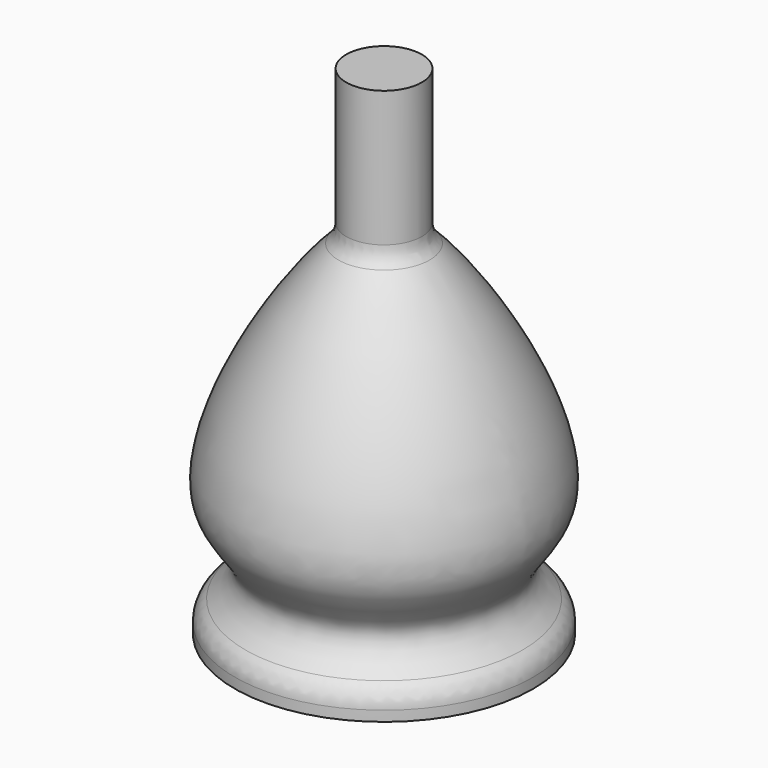
from build123d import *

# Parameters (mm, degrees)
F2_R     = 5.08
F3_DEPTH = 30.48
F4_R     = 5.08


with BuildPart() as f1:
    # F0 (on Front) → F1 (revolve)
    with BuildSketch(Plane.XZ):
        with BuildLine():
            add(Edge.make_bspline(
                [(8.1309033558, 71.12), (7.9376181833, 71.2042943301), (7.8304224666, 71.1715075808), (7.7253221534, 71.12)],
                knots=[0.9636093673, 0.9636093673, 0.9636093673, 0.9636093673, 1, 1, 1, 1], degree=3))
            Line((7.7253221534, 71.12), (8.1309033558, 71.12))
        make_face()
        with BuildLine():
            Line((0, 71.12), (0, 0))
            Line((0, 0), (30.48, 0))
            Line((30.48, 0), (30.48, 5.08))
            add(Edge.make_bspline(
                [(30.48, 5.08), (27.3303148752, 6.3370296731), (20.5275560182, 13.3757986931), (36.6852035847, 23.8800059507), (21.5393568197, 56.9061702589), (9.4088823722, 70.5626557213), (8.1309033558, 71.12)],
                knots=[0, 0, 0, 0, 0.1775699554, 0.3846763281, 0.7229987487, 0.9636093673, 0.9636093673, 0.9636093673, 0.9636093673], degree=3))
            Line((8.1309033558, 71.12), (7.7253221534, 71.12))
            Line((7.7253221534, 71.12), (0, 71.12))
        make_face()
    revolve(axis=Axis((0, 0, 35.56), (0, 0, 1)))

    # F2
    f2_edges = [f1.edges().sort_by_distance(p)[0] for p in [
        (-30.48, 0, 5.08),
    ]]
    fillet(f2_edges, radius=F2_R)

    # F3 (add): a face of the model
    f3_faces = [f1.faces().sort_by_distance(p)[0] for p in [
        (0, 0, 71.12),
    ]]
    extrude(f3_faces, amount=F3_DEPTH)

    # F4
    f4_edges = [f1.edges().sort_by_distance(p)[0] for p in [
        (-7.725322, 0, 71.12),
    ]]
    fillet(f4_edges, radius=F4_R)


solid = f1.part
